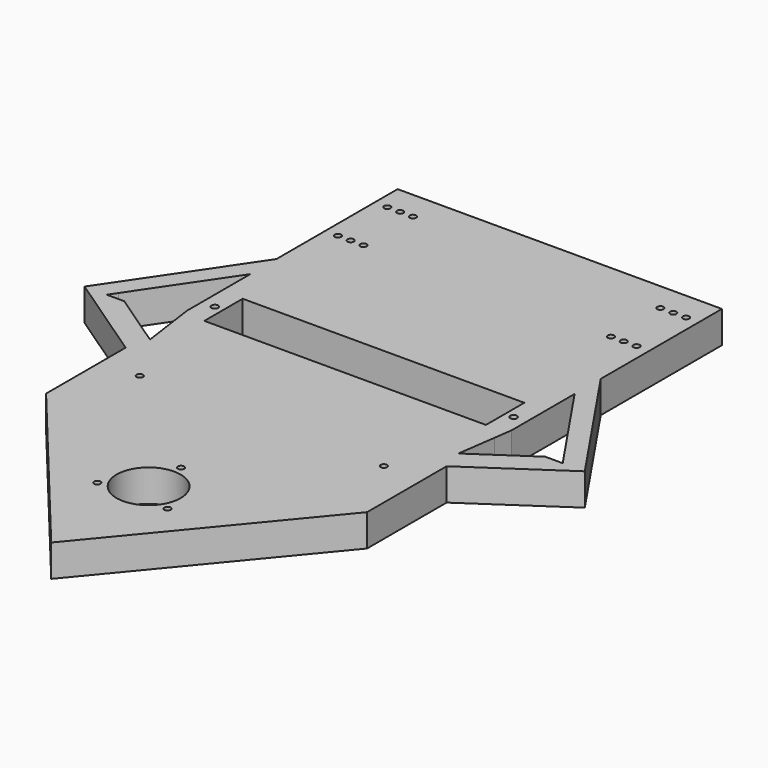
from build123d import *

# Parameters (mm, degrees)
F0_R      = 1.5
F1_DEPTH  = 5
F2_DEPTH  = 25
F3_DEPTH  = 25
F5_DEPTH  = 93
F6_DEPTH  = 8
F8_DEPTH  = 126
F7_R      = 1.5
F9_DEPTH  = 51.9
F10_DEPTH = 5
F11_DEPTH = 123
F12_DEPTH = 10


with BuildPart() as f1:
    # F0 (on Top) → F1 (new body)
    with BuildSketch(Plane.XY):
        Polygon((76, 118.35680902), (76, 131.8702431194), (-76, 131.8702431194), (-76, 60.855999589), (-76, 45.5639077712), (-76, 8.6270240996), (-74.7927818864, 0), (0, 0), (74.7927818864, 0), (76, 8.6270240996), (76, 45.5639077712), (76, 60.855999589), align=None)
        with Locations((-70, 89.35680902)):
            Circle(F0_R, mode=Mode.SUBTRACT)
        with Locations((-64, 89.35680902)):
            Circle(F0_R, mode=Mode.SUBTRACT)
        with Locations((-70, 118.35680902)):
            Circle(F0_R, mode=Mode.SUBTRACT)
        with Locations((-64, 118.35680902)):
            Circle(F0_R, mode=Mode.SUBTRACT)
        with Locations((-58, 89.35680902)):
            Circle(F0_R, mode=Mode.SUBTRACT)
        with Locations((-58, 118.35680902)):
            Circle(F0_R, mode=Mode.SUBTRACT)
        with Locations((58, 89.35680902)):
            Circle(F0_R, mode=Mode.SUBTRACT)
        with Locations((58, 118.35680902)):
            Circle(F0_R, mode=Mode.SUBTRACT)
        with Locations((64, 89.35680902)):
            Circle(F0_R, mode=Mode.SUBTRACT)
        with Locations((70, 89.35680902)):
            Circle(F0_R, mode=Mode.SUBTRACT)
        with Locations((64, 118.35680902)):
            Circle(F0_R, mode=Mode.SUBTRACT)
        with Locations((70, 118.35680902)):
            Circle(F0_R, mode=Mode.SUBTRACT)
        Polygon((-76, 45.5639077712), (-76, 60.855999589), (-117.2245144844, 0), (-106.865485549, 0), (-104.2798289376, 3.8169695785), align=None)
        Polygon((117.2245144844, 0), (76, 60.855999589), (76, 45.5639077712), (87.8824198706, 28.022972534), (104.2798289376, 3.8169695785), (106.865485549, 0), align=None)
        with BuildLine():
            Line((-106.865485549, 0), (-117.2245144844, 0))
            Line((-117.2245144844, 0), (-75.2239967593, -28.4516064646))
            Line((-75.2239967593, -28.4516064646), (-75.2239967593, -75.0488862395))
            Line((-75.2239967593, -75.0488862395), (0, -166.0707890987))
            Line((0, -166.0707890987), (0, -124.006434679))
            ThreePointArc((0, -124.006434679), (-15, -109.006434679), (0, -94.006434679))
            Line((0, -94.006434679), (0, -91.506434679))
            ThreePointArc((0, -91.506434679), (-1.5, -90.006434679), (0, -88.506434679))
            Line((0, -88.506434679), (0, -73.5419392586))
            Line((0, -73.5419392586), (0, 0))
            Line((0, 0), (-74.7927818864, 0))
            Line((-74.7927818864, 0), (-72.2949617347, -17.8499265401))
            Line((-72.2949617347, -17.8499265401), (-98.6451840666, 0))
            Line((-98.6451840666, 0), (-106.865485549, 0))
        make_face()
        with Locations((-16.4544826719, -118.506434679)):
            Circle(F0_R, mode=Mode.SUBTRACT)
        with BuildLine():
            Line((75.2239967593, -28.4516064646), (117.2245144844, 0))
            Line((117.2245144844, 0), (106.865485549, 0))
            Line((106.865485549, 0), (98.6451840666, 0))
            Line((98.6451840666, 0), (72.2949617347, -17.8499265401))
            Line((72.2949617347, -17.8499265401), (74.7927818864, 0))
            Line((74.7927818864, 0), (0, 0))
            Line((0, 0), (0, -73.5419392586))
            Line((0, -73.5419392586), (0, -88.506434679))
            ThreePointArc((0, -88.506434679), (1.0606601718, -88.9457745073), (1.5, -90.006434679))
            ThreePointArc((1.5, -90.006434679), (1.0606601718, -91.0670948508), (0, -91.506434679))
            Line((0, -91.506434679), (0, -94.006434679))
            ThreePointArc((0, -94.006434679), (10.6066017178, -98.3998329612), (15, -109.006434679))
            ThreePointArc((15, -109.006434679), (10.6066017178, -119.6130363968), (0, -124.006434679))
            Line((0, -124.006434679), (0, -166.0707890987))
            Line((0, -166.0707890987), (75.2239967593, -75.0488862395))
            Line((75.2239967593, -75.0488862395), (75.2239967593, -28.4516064646))
        make_face()
        with Locations((16.4544826719, -118.506434679)):
            Circle(F0_R, mode=Mode.SUBTRACT)
    extrude(amount=F1_DEPTH)

    # F0 (on Top) → F2 (join)
    with BuildSketch(Plane.XY):
        Polygon((76, 118.35680902), (76, 131.8702431194), (-76, 131.8702431194), (-76, 60.855999589), (-76, 45.5639077712), (-76, 8.6270240996), (-74.7927818864, 0), (0, 0), (74.7927818864, 0), (76, 8.6270240996), (76, 45.5639077712), (76, 60.855999589), align=None)
        with Locations((-70, 89.35680902)):
            Circle(F0_R, mode=Mode.SUBTRACT)
        with Locations((-64, 89.35680902)):
            Circle(F0_R, mode=Mode.SUBTRACT)
        with Locations((-70, 118.35680902)):
            Circle(F0_R, mode=Mode.SUBTRACT)
        with Locations((-64, 118.35680902)):
            Circle(F0_R, mode=Mode.SUBTRACT)
        with Locations((-58, 89.35680902)):
            Circle(F0_R, mode=Mode.SUBTRACT)
        with Locations((-58, 118.35680902)):
            Circle(F0_R, mode=Mode.SUBTRACT)
        with Locations((58, 89.35680902)):
            Circle(F0_R, mode=Mode.SUBTRACT)
        with Locations((58, 118.35680902)):
            Circle(F0_R, mode=Mode.SUBTRACT)
        with Locations((64, 89.35680902)):
            Circle(F0_R, mode=Mode.SUBTRACT)
        with Locations((70, 89.35680902)):
            Circle(F0_R, mode=Mode.SUBTRACT)
        with Locations((64, 118.35680902)):
            Circle(F0_R, mode=Mode.SUBTRACT)
        with Locations((70, 118.35680902)):
            Circle(F0_R, mode=Mode.SUBTRACT)
        Polygon((-76, 45.5639077712), (-76, 60.855999589), (-117.2245144844, 0), (-106.865485549, 0), (-104.2798289376, 3.8169695785), align=None)
        Polygon((117.2245144844, 0), (76, 60.855999589), (76, 45.5639077712), (87.8824198706, 28.022972534), (104.2798289376, 3.8169695785), (106.865485549, 0), align=None)
        with BuildLine():
            Line((-106.865485549, 0), (-117.2245144844, 0))
            Line((-117.2245144844, 0), (-75.2239967593, -28.4516064646))
            Line((-75.2239967593, -28.4516064646), (-75.2239967593, -75.0488862395))
            Line((-75.2239967593, -75.0488862395), (0, -166.0707890987))
            Line((0, -166.0707890987), (0, -124.006434679))
            ThreePointArc((0, -124.006434679), (-15, -109.006434679), (0, -94.006434679))
            Line((0, -94.006434679), (0, -91.506434679))
            ThreePointArc((0, -91.506434679), (-1.5, -90.006434679), (0, -88.506434679))
            Line((0, -88.506434679), (0, -73.5419392586))
            Line((0, -73.5419392586), (0, 0))
            Line((0, 0), (-74.7927818864, 0))
            Line((-74.7927818864, 0), (-72.2949617347, -17.8499265401))
            Line((-72.2949617347, -17.8499265401), (-98.6451840666, 0))
            Line((-98.6451840666, 0), (-106.865485549, 0))
        make_face()
        with Locations((-16.4544826719, -118.506434679)):
            Circle(F0_R, mode=Mode.SUBTRACT)
        with BuildLine():
            Line((75.2239967593, -28.4516064646), (117.2245144844, 0))
            Line((117.2245144844, 0), (106.865485549, 0))
            Line((106.865485549, 0), (98.6451840666, 0))
            Line((98.6451840666, 0), (72.2949617347, -17.8499265401))
            Line((72.2949617347, -17.8499265401), (74.7927818864, 0))
            Line((74.7927818864, 0), (0, 0))
            Line((0, 0), (0, -73.5419392586))
            Line((0, -73.5419392586), (0, -88.506434679))
            ThreePointArc((0, -88.506434679), (1.0606601718, -88.9457745073), (1.5, -90.006434679))
            ThreePointArc((1.5, -90.006434679), (1.0606601718, -91.0670948508), (0, -91.506434679))
            Line((0, -91.506434679), (0, -94.006434679))
            ThreePointArc((0, -94.006434679), (10.6066017178, -98.3998329612), (15, -109.006434679))
            ThreePointArc((15, -109.006434679), (10.6066017178, -119.6130363968), (0, -124.006434679))
            Line((0, -124.006434679), (0, -166.0707890987))
            Line((0, -166.0707890987), (75.2239967593, -75.0488862395))
            Line((75.2239967593, -75.0488862395), (75.2239967593, -28.4516064646))
        make_face()
        with Locations((16.4544826719, -118.506434679)):
            Circle(F0_R, mode=Mode.SUBTRACT)
    extrude(amount=F2_DEPTH)

    # F0 (on Top) → F3 (join)
    with BuildSketch(Plane.XY):
        Polygon((76, 118.35680902), (76, 131.8702431194), (-76, 131.8702431194), (-76, 60.855999589), (-76, 45.5639077712), (-76, 8.6270240996), (-74.7927818864, 0), (0, 0), (74.7927818864, 0), (76, 8.6270240996), (76, 45.5639077712), (76, 60.855999589), align=None)
        with Locations((-70, 89.35680902)):
            Circle(F0_R, mode=Mode.SUBTRACT)
        with Locations((-64, 89.35680902)):
            Circle(F0_R, mode=Mode.SUBTRACT)
        with Locations((-70, 118.35680902)):
            Circle(F0_R, mode=Mode.SUBTRACT)
        with Locations((-64, 118.35680902)):
            Circle(F0_R, mode=Mode.SUBTRACT)
        with Locations((-58, 89.35680902)):
            Circle(F0_R, mode=Mode.SUBTRACT)
        with Locations((-58, 118.35680902)):
            Circle(F0_R, mode=Mode.SUBTRACT)
        with Locations((58, 89.35680902)):
            Circle(F0_R, mode=Mode.SUBTRACT)
        with Locations((58, 118.35680902)):
            Circle(F0_R, mode=Mode.SUBTRACT)
        with Locations((64, 89.35680902)):
            Circle(F0_R, mode=Mode.SUBTRACT)
        with Locations((70, 89.35680902)):
            Circle(F0_R, mode=Mode.SUBTRACT)
        with Locations((64, 118.35680902)):
            Circle(F0_R, mode=Mode.SUBTRACT)
        with Locations((70, 118.35680902)):
            Circle(F0_R, mode=Mode.SUBTRACT)
        Polygon((-76, 45.5639077712), (-76, 60.855999589), (-117.2245144844, 0), (-106.865485549, 0), (-104.2798289376, 3.8169695785), align=None)
        Polygon((117.2245144844, 0), (76, 60.855999589), (76, 45.5639077712), (87.8824198706, 28.022972534), (104.2798289376, 3.8169695785), (106.865485549, 0), align=None)
        with BuildLine():
            Line((-106.865485549, 0), (-117.2245144844, 0))
            Line((-117.2245144844, 0), (-75.2239967593, -28.4516064646))
            Line((-75.2239967593, -28.4516064646), (-75.2239967593, -75.0488862395))
            Line((-75.2239967593, -75.0488862395), (0, -166.0707890987))
            Line((0, -166.0707890987), (0, -124.006434679))
            ThreePointArc((0, -124.006434679), (-15, -109.006434679), (0, -94.006434679))
            Line((0, -94.006434679), (0, -91.506434679))
            ThreePointArc((0, -91.506434679), (-1.5, -90.006434679), (0, -88.506434679))
            Line((0, -88.506434679), (0, -73.5419392586))
            Line((0, -73.5419392586), (0, 0))
            Line((0, 0), (-74.7927818864, 0))
            Line((-74.7927818864, 0), (-72.2949617347, -17.8499265401))
            Line((-72.2949617347, -17.8499265401), (-98.6451840666, 0))
            Line((-98.6451840666, 0), (-106.865485549, 0))
        make_face()
        with Locations((-16.4544826719, -118.506434679)):
            Circle(F0_R, mode=Mode.SUBTRACT)
        with BuildLine():
            Line((75.2239967593, -28.4516064646), (117.2245144844, 0))
            Line((117.2245144844, 0), (106.865485549, 0))
            Line((106.865485549, 0), (98.6451840666, 0))
            Line((98.6451840666, 0), (72.2949617347, -17.8499265401))
            Line((72.2949617347, -17.8499265401), (74.7927818864, 0))
            Line((74.7927818864, 0), (0, 0))
            Line((0, 0), (0, -73.5419392586))
            Line((0, -73.5419392586), (0, -88.506434679))
            ThreePointArc((0, -88.506434679), (1.0606601718, -88.9457745073), (1.5, -90.006434679))
            ThreePointArc((1.5, -90.006434679), (1.0606601718, -91.0670948508), (0, -91.506434679))
            Line((0, -91.506434679), (0, -94.006434679))
            ThreePointArc((0, -94.006434679), (10.6066017178, -98.3998329612), (15, -109.006434679))
            ThreePointArc((15, -109.006434679), (10.6066017178, -119.6130363968), (0, -124.006434679))
            Line((0, -124.006434679), (0, -166.0707890987))
            Line((0, -166.0707890987), (75.2239967593, -75.0488862395))
            Line((75.2239967593, -75.0488862395), (75.2239967593, -28.4516064646))
        make_face()
        with Locations((16.4544826719, -118.506434679)):
            Circle(F0_R, mode=Mode.SUBTRACT)
    extrude(amount=F3_DEPTH)

    # F4 (on Top) → F5 (cut)
    with BuildSketch(Plane.XY):
        Polygon((-66, 28.6083016545), (-66, 6.1162575148), (-49.9165579677, 6.1162575148), (66, 6.1162575148), (66, 28.6083016545), align=None)
        with BuildLine():
            ThreePointArc((70, 15.7622795846), (71.1313708499, 16.2309087347), (71.6, 17.3622795846))
            ThreePointArc((71.6, 17.3622795846), (68.8686291501, 18.4936504345), (70, 15.7622795846))
        make_face()
        with BuildLine():
            ThreePointArc((-70, 15.7120144755), (-68.8686291501, 16.1806436256), (-68.4, 17.3120144755))
            ThreePointArc((-68.4, 17.3120144755), (-71.1313708499, 18.4433853254), (-70, 15.7120144755))
        make_face()
    extrude(amount=F5_DEPTH, mode=Mode.SUBTRACT)

    # F0 (on Top) → F6 (join)
    with BuildSketch(Plane.XY):
        Polygon((76, 118.35680902), (76, 131.8702431194), (-76, 131.8702431194), (-76, 60.855999589), (-76, 45.5639077712), (-76, 8.6270240996), (-74.7927818864, 0), (0, 0), (74.7927818864, 0), (76, 8.6270240996), (76, 45.5639077712), (76, 60.855999589), align=None)
        with Locations((-70, 89.35680902)):
            Circle(F0_R, mode=Mode.SUBTRACT)
        with Locations((-64, 89.35680902)):
            Circle(F0_R, mode=Mode.SUBTRACT)
        with Locations((-70, 118.35680902)):
            Circle(F0_R, mode=Mode.SUBTRACT)
        with Locations((-64, 118.35680902)):
            Circle(F0_R, mode=Mode.SUBTRACT)
        with Locations((-58, 89.35680902)):
            Circle(F0_R, mode=Mode.SUBTRACT)
        with Locations((-58, 118.35680902)):
            Circle(F0_R, mode=Mode.SUBTRACT)
        with Locations((58, 89.35680902)):
            Circle(F0_R, mode=Mode.SUBTRACT)
        with Locations((58, 118.35680902)):
            Circle(F0_R, mode=Mode.SUBTRACT)
        with Locations((64, 89.35680902)):
            Circle(F0_R, mode=Mode.SUBTRACT)
        with Locations((70, 89.35680902)):
            Circle(F0_R, mode=Mode.SUBTRACT)
        with Locations((64, 118.35680902)):
            Circle(F0_R, mode=Mode.SUBTRACT)
        with Locations((70, 118.35680902)):
            Circle(F0_R, mode=Mode.SUBTRACT)
        Polygon((-76, 45.5639077712), (-76, 60.855999589), (-117.2245144844, 0), (-106.865485549, 0), (-104.2798289376, 3.8169695785), align=None)
        Polygon((117.2245144844, 0), (76, 60.855999589), (76, 45.5639077712), (87.8824198706, 28.022972534), (104.2798289376, 3.8169695785), (106.865485549, 0), align=None)
        with BuildLine():
            Line((-106.865485549, 0), (-117.2245144844, 0))
            Line((-117.2245144844, 0), (-75.2239967593, -28.4516064646))
            Line((-75.2239967593, -28.4516064646), (-75.2239967593, -75.0488862395))
            Line((-75.2239967593, -75.0488862395), (0, -166.0707890987))
            Line((0, -166.0707890987), (0, -124.006434679))
            ThreePointArc((0, -124.006434679), (-15, -109.006434679), (0, -94.006434679))
            Line((0, -94.006434679), (0, -91.506434679))
            ThreePointArc((0, -91.506434679), (-1.5, -90.006434679), (0, -88.506434679))
            Line((0, -88.506434679), (0, -73.5419392586))
            Line((0, -73.5419392586), (0, 0))
            Line((0, 0), (-74.7927818864, 0))
            Line((-74.7927818864, 0), (-72.2949617347, -17.8499265401))
            Line((-72.2949617347, -17.8499265401), (-98.6451840666, 0))
            Line((-98.6451840666, 0), (-106.865485549, 0))
        make_face()
        with Locations((-16.4544826719, -118.506434679)):
            Circle(F0_R, mode=Mode.SUBTRACT)
        with BuildLine():
            Line((75.2239967593, -28.4516064646), (117.2245144844, 0))
            Line((117.2245144844, 0), (106.865485549, 0))
            Line((106.865485549, 0), (98.6451840666, 0))
            Line((98.6451840666, 0), (72.2949617347, -17.8499265401))
            Line((72.2949617347, -17.8499265401), (74.7927818864, 0))
            Line((74.7927818864, 0), (0, 0))
            Line((0, 0), (0, -73.5419392586))
            Line((0, -73.5419392586), (0, -88.506434679))
            ThreePointArc((0, -88.506434679), (1.0606601718, -88.9457745073), (1.5, -90.006434679))
            ThreePointArc((1.5, -90.006434679), (1.0606601718, -91.0670948508), (0, -91.506434679))
            Line((0, -91.506434679), (0, -94.006434679))
            ThreePointArc((0, -94.006434679), (10.6066017178, -98.3998329612), (15, -109.006434679))
            ThreePointArc((15, -109.006434679), (10.6066017178, -119.6130363968), (0, -124.006434679))
            Line((0, -124.006434679), (0, -166.0707890987))
            Line((0, -166.0707890987), (75.2239967593, -75.0488862395))
            Line((75.2239967593, -75.0488862395), (75.2239967593, -28.4516064646))
        make_face()
        with Locations((16.4544826719, -118.506434679)):
            Circle(F0_R, mode=Mode.SUBTRACT)
    extrude(amount=F6_DEPTH)

    # F4 (on Top) → F8 (cut)
    with BuildSketch(Plane.XY):
        Polygon((-66, 28.6083016545), (-66, 6.1162575148), (-49.9165579677, 6.1162575148), (66, 6.1162575148), (66, 28.6083016545), align=None)
        with BuildLine():
            ThreePointArc((70, 15.7622795846), (71.1313708499, 16.2309087347), (71.6, 17.3622795846))
            ThreePointArc((71.6, 17.3622795846), (68.8686291501, 18.4936504345), (70, 15.7622795846))
        make_face()
        with BuildLine():
            ThreePointArc((-70, 15.7120144755), (-68.8686291501, 16.1806436256), (-68.4, 17.3120144755))
            ThreePointArc((-68.4, 17.3120144755), (-71.1313708499, 18.4433853254), (-70, 15.7120144755))
        make_face()
    extrude(amount=F8_DEPTH, mode=Mode.SUBTRACT)

    # F7 (on Top) → F9 (cut)
    with BuildSketch(Plane.XY):
        with BuildLine():
            ThreePointArc((-57.2169274092, -41.1575653255), (-58.277587581, -43.7182254973), (-55.7169274092, -42.6575653255))
            ThreePointArc((-55.7169274092, -42.6575653255), (-56.1562672374, -41.5969051537), (-57.2169274092, -41.1575653255))
        make_face()
        with Locations((57.2169274092, -42.6575653255)):
            Circle(F7_R)
    extrude(amount=F9_DEPTH, mode=Mode.SUBTRACT)

    # F0 (on Top) → F10 (join)
    with BuildSketch(Plane.XY):
        Polygon((76, 118.35680902), (76, 131.8702431194), (-76, 131.8702431194), (-76, 60.855999589), (-76, 45.5639077712), (-76, 8.6270240996), (-74.7927818864, 0), (0, 0), (74.7927818864, 0), (76, 8.6270240996), (76, 45.5639077712), (76, 60.855999589), align=None)
        with Locations((-70, 89.35680902)):
            Circle(F0_R, mode=Mode.SUBTRACT)
        with Locations((-64, 89.35680902)):
            Circle(F0_R, mode=Mode.SUBTRACT)
        with Locations((-70, 118.35680902)):
            Circle(F0_R, mode=Mode.SUBTRACT)
        with Locations((-64, 118.35680902)):
            Circle(F0_R, mode=Mode.SUBTRACT)
        with Locations((-58, 89.35680902)):
            Circle(F0_R, mode=Mode.SUBTRACT)
        with Locations((-58, 118.35680902)):
            Circle(F0_R, mode=Mode.SUBTRACT)
        with Locations((58, 89.35680902)):
            Circle(F0_R, mode=Mode.SUBTRACT)
        with Locations((58, 118.35680902)):
            Circle(F0_R, mode=Mode.SUBTRACT)
        with Locations((64, 89.35680902)):
            Circle(F0_R, mode=Mode.SUBTRACT)
        with Locations((70, 89.35680902)):
            Circle(F0_R, mode=Mode.SUBTRACT)
        with Locations((64, 118.35680902)):
            Circle(F0_R, mode=Mode.SUBTRACT)
        with Locations((70, 118.35680902)):
            Circle(F0_R, mode=Mode.SUBTRACT)
        Polygon((-76, 45.5639077712), (-76, 60.855999589), (-117.2245144844, 0), (-106.865485549, 0), (-104.2798289376, 3.8169695785), align=None)
        Polygon((117.2245144844, 0), (76, 60.855999589), (76, 45.5639077712), (87.8824198706, 28.022972534), (104.2798289376, 3.8169695785), (106.865485549, 0), align=None)
        with BuildLine():
            Line((-106.865485549, 0), (-117.2245144844, 0))
            Line((-117.2245144844, 0), (-75.2239967593, -28.4516064646))
            Line((-75.2239967593, -28.4516064646), (-75.2239967593, -75.0488862395))
            Line((-75.2239967593, -75.0488862395), (0, -166.0707890987))
            Line((0, -166.0707890987), (0, -124.006434679))
            ThreePointArc((0, -124.006434679), (-15, -109.006434679), (0, -94.006434679))
            Line((0, -94.006434679), (0, -91.506434679))
            ThreePointArc((0, -91.506434679), (-1.5, -90.006434679), (0, -88.506434679))
            Line((0, -88.506434679), (0, -73.5419392586))
            Line((0, -73.5419392586), (0, 0))
            Line((0, 0), (-74.7927818864, 0))
            Line((-74.7927818864, 0), (-72.2949617347, -17.8499265401))
            Line((-72.2949617347, -17.8499265401), (-98.6451840666, 0))
            Line((-98.6451840666, 0), (-106.865485549, 0))
        make_face()
        with Locations((-16.4544826719, -118.506434679)):
            Circle(F0_R, mode=Mode.SUBTRACT)
        with BuildLine():
            Line((75.2239967593, -28.4516064646), (117.2245144844, 0))
            Line((117.2245144844, 0), (106.865485549, 0))
            Line((106.865485549, 0), (98.6451840666, 0))
            Line((98.6451840666, 0), (72.2949617347, -17.8499265401))
            Line((72.2949617347, -17.8499265401), (74.7927818864, 0))
            Line((74.7927818864, 0), (0, 0))
            Line((0, 0), (0, -73.5419392586))
            Line((0, -73.5419392586), (0, -88.506434679))
            ThreePointArc((0, -88.506434679), (1.0606601718, -88.9457745073), (1.5, -90.006434679))
            ThreePointArc((1.5, -90.006434679), (1.0606601718, -91.0670948508), (0, -91.506434679))
            Line((0, -91.506434679), (0, -94.006434679))
            ThreePointArc((0, -94.006434679), (10.6066017178, -98.3998329612), (15, -109.006434679))
            ThreePointArc((15, -109.006434679), (10.6066017178, -119.6130363968), (0, -124.006434679))
            Line((0, -124.006434679), (0, -166.0707890987))
            Line((0, -166.0707890987), (75.2239967593, -75.0488862395))
            Line((75.2239967593, -75.0488862395), (75.2239967593, -28.4516064646))
        make_face()
        with Locations((16.4544826719, -118.506434679)):
            Circle(F0_R, mode=Mode.SUBTRACT)
    extrude(amount=F10_DEPTH)

    # F11 (cut): faces of the model
    f11_faces = [f1.faces().sort_by_distance(p)[0] for p in [
        (70, 17.3622795846, 5),
        (0, 17.3622795846, 5),
        (-70, 17.3120144755, 5),
    ]]
    extrude(f11_faces, amount=-F11_DEPTH, mode=Mode.SUBTRACT)

    # F12 (cut): a face of the model
    f12_faces = [f1.faces().sort_by_distance(p)[0] for p in [
        (0, 5.9527027765, 0),
    ]]
    extrude(f12_faces, amount=-F12_DEPTH, mode=Mode.SUBTRACT)


solid = f1.part
